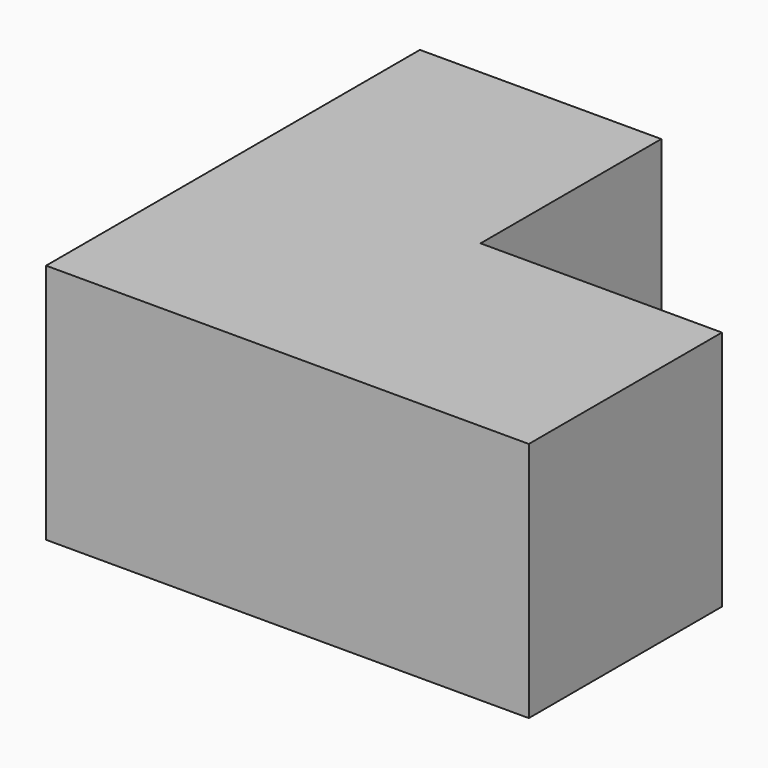
from build123d import *

# Parameters (mm, degrees)
F1_W     = 127
F1_H     = 127
F2_DEPTH = 127
F3_W     = 127
F3_H     = 127
F4_DEPTH = 245.872


# Not quite as in the source:
# - a variable given as a bare number and used for a length is read in inches; the dataset says mm whatever the document's units were


with BuildPart() as f2:
    # F1 (on Front) → F2 (new body)
    with BuildSketch(Plane.XZ):
        with Locations((-59.2341877744, -35.8161340777)):
            Rectangle(F1_W, F1_H)
    extrude(amount=F2_DEPTH)

    # F3 (on face) → F4 (join)
    with BuildSketch(Plane.XZ.offset(127)):
        with Locations((-186.2341877744, -35.8161340777)):
            Rectangle(F3_W, F3_H)
    extrude(amount=-F4_DEPTH)


solid = f2.part
